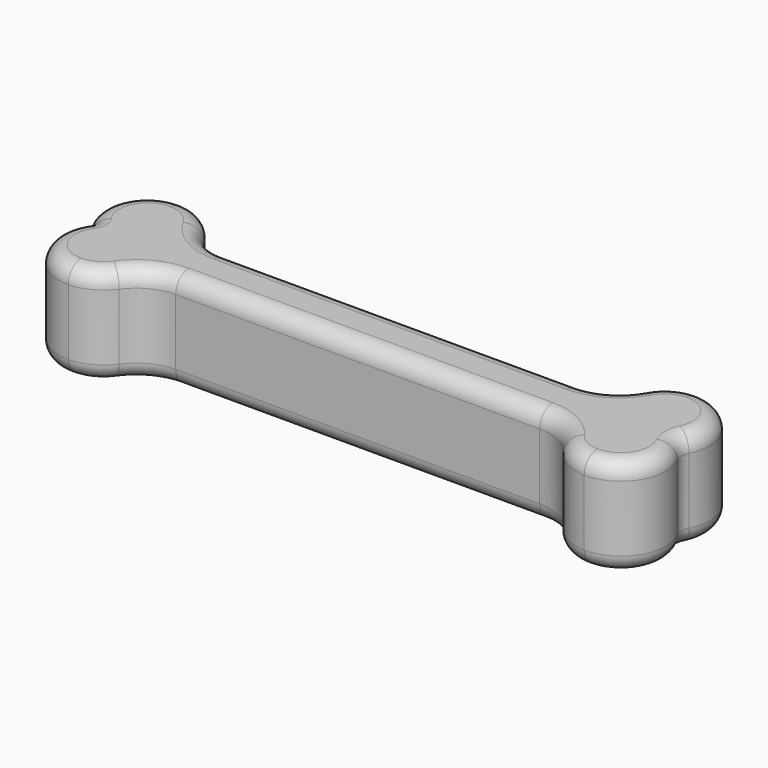
from build123d import *

# Parameters (mm, degrees)
F1_DEPTH = 12.7
F2_SCALE = 3
F3_R     = 6.35


with BuildPart() as f1:
    # F0 (on Top) → F1 (new body)
    with BuildSketch(Plane.XY):
        with BuildLine():
            Line((22.650744566, 7.190999575), (0, 7.190999575))
            Line((0, 7.190999575), (-22.650744566, 7.190999575))
            ThreePointArc((-22.650744566, 7.190999575), (-25.858668803, 8.0608789477), (-28.1876931588, 10.432189468))
            ThreePointArc((-28.1876931588, 10.432189468), (-30.2562615135, 12.5550773402), (-33.1075824797, 13.3647666037))
            ThreePointArc((-33.1075824797, 13.3647666037), (-38.2854180827, 10.2927602437), (-37.8803053875, 4.2858402083))
            ThreePointArc((-37.8803053875, 4.2858402083), (-37.833228654, 4.137603143), (-37.8813892603, 3.9897146635))
            ThreePointArc((-37.8813892603, 3.9897146635), (-38.3233098407, -2.0656424962), (-33.1075824797, -5.1735086816))
            ThreePointArc((-33.1075824797, -5.1735086816), (-30.5246049962, -4.5182552091), (-28.51033034, -2.7735983939))
            ThreePointArc((-28.51033034, -2.7735983939), (-26.2523403785, -0.8333702379), (-23.3582126367, -0.1354959101))
            Line((-23.3582126367, -0.1354959101), (0, -0.1354959101))
            Line((0, -0.1354959101), (23.3582126367, -0.1354959101))
            ThreePointArc((23.3582126367, -0.1354959101), (26.2523403785, -0.8333702379), (28.51033034, -2.7735983939))
            ThreePointArc((28.51033034, -2.7735983939), (30.5246049962, -4.5182552091), (33.1075824797, -5.1735086816))
            ThreePointArc((33.1075824797, -5.1735086816), (38.3652517819, -1.983544068), (37.7709929375, 4.1373886349))
            ThreePointArc((37.7709929375, 4.1373886349), (38.3276553946, 10.2108253524), (33.1075824797, 13.3647666037))
            ThreePointArc((33.1075824797, 13.3647666037), (30.2562615135, 12.5550773402), (28.1876931588, 10.432189468))
            ThreePointArc((28.1876931588, 10.432189468), (25.858668803, 8.0608789477), (22.650744566, 7.190999575))
        make_face()
    extrude(amount=F1_DEPTH)


with BuildPart() as f1_1:
    # F2: moved
    add(f1.part.scale(F2_SCALE))

    # F3
    f3_edges = [f1_1.edges().sort_by_distance(p)[0] for p in [
        (77.576006, 24.182637, 0),
        (0, 21.572999, 0),
        (-77.576006, 24.182637, 0),
        (-108.828758, 37.41586, 0),
        (-113.499686, 12.412809, 0),
        (-109.740982, -12.244098, 0),
        (-78.757021, -2.500111, 0),
        (0, -0.406488, 0),
        (78.757021, -2.500111, 0),
        (109.96395, -12.080456, 0),
        (109.061108, 37.265895, 0),
        (113.312979, 12.412166, 19.05),
        (77.576006, 24.182637, 38.1),
        (0, 21.572999, 38.1),
        (-77.576006, 24.182637, 38.1),
        (-108.828758, 37.41586, 38.1),
        (-113.499686, 12.412809, 38.1),
        (-109.740982, -12.244098, 38.1),
        (-78.757021, -2.500111, 38.1),
        (0, -0.406488, 38.1),
        (78.757021, -2.500111, 38.1),
        (109.96395, -12.080456, 38.1),
        (109.061108, 37.265895, 38.1),
    ]]
    fillet(f3_edges, radius=F3_R)


solid = f1_1.part
